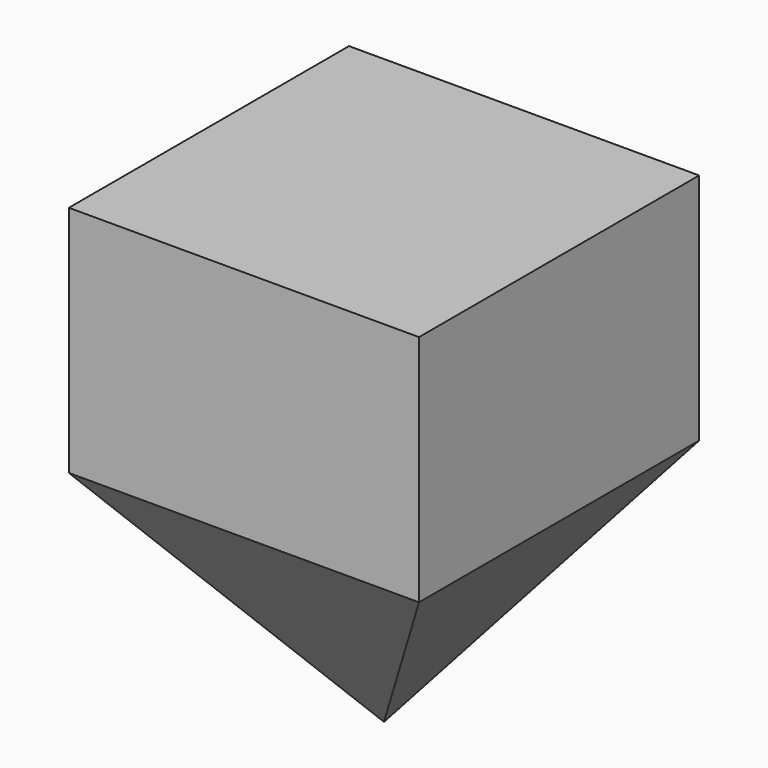
from build123d import *

# Parameters (mm, degrees)
F0_W     = 38.1
F0_H     = 38.1
F1_DEPTH = 50.8
F2_SIZE2 = 25.39999
F2_SIZE  = 19.04999


# Not quite as in the source:
# - a fillet or chamfer is up to 0.001 mm smaller than in the source, because OpenCascade refuses the exact size


with BuildPart() as f1:
    # F0 (on Top) → F1 (new body)
    with BuildSketch(Plane.XY):
        Rectangle(F0_W, F0_H)
    extrude(amount=F1_DEPTH)

    # F2 (size 19.05 and 25.4 in the source; OpenCascade refuses exactly that, so slightly less here)
    f2_edges = [f1.edges().sort_by_distance(p)[0] for p in [
        (0, 19.05, 0),
        (-19.05, 0, 0),
        (0, -19.05, 0),
        (19.05, 0, 0),
    ]]
    f2_side = f1.faces().sort_by_distance((0, 0, 0))[0]
    chamfer(f2_edges, length=F2_SIZE, length2=F2_SIZE2, reference=f2_side)


solid = f1.part
